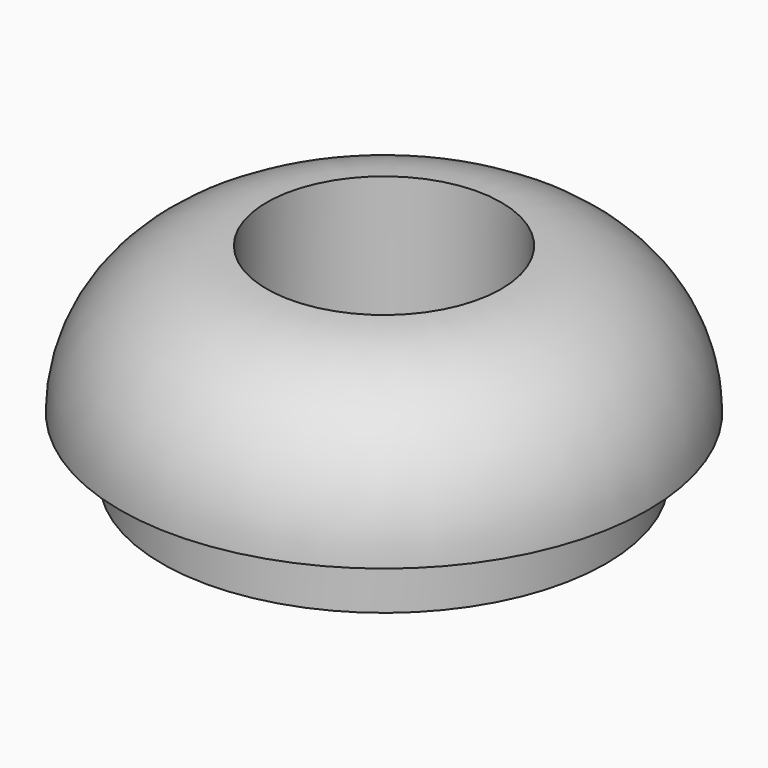
from build123d import *

# Parameters (mm, degrees)
F0_R        = 12.4
F0_R_2      = 6.55
F1_DEPTH    = 3.4
F0_R_3      = 14.75
F1_FACE_R   = 12.4
F1_FACE_R_2 = 6.55
F2_DEPTH    = 8.2
F3_R        = 8.19999


# Not quite as in the source:
# - a fillet or chamfer is up to 0.001 mm smaller than in the source, because OpenCascade refuses the exact size


with BuildPart() as f1:
    # F0 (on Top) → F1 (new body)
    with BuildSketch(Plane.XY):
        Circle(F0_R)
        Circle(F0_R_2, mode=Mode.SUBTRACT)
    extrude(amount=-F1_DEPTH)

    # F0 (on Top) + F1_face (on face) → F2 (join)
    with BuildSketch(Plane.XY):
        Circle(F0_R_3)
        Circle(F0_R, mode=Mode.SUBTRACT)
    with BuildSketch(Plane.XY):
        Circle(F1_FACE_R)
        Circle(F1_FACE_R_2, mode=Mode.SUBTRACT)
    extrude(amount=F2_DEPTH)

    # F3 (radius 8.2 in the source; OpenCascade refuses exactly that, so slightly less here)
    f3_edges = [f1.edges().sort_by_distance(p)[0] for p in [
        (-14.75, 0, 8.2),
    ]]
    fillet(f3_edges, radius=F3_R)


solid = f1.part
